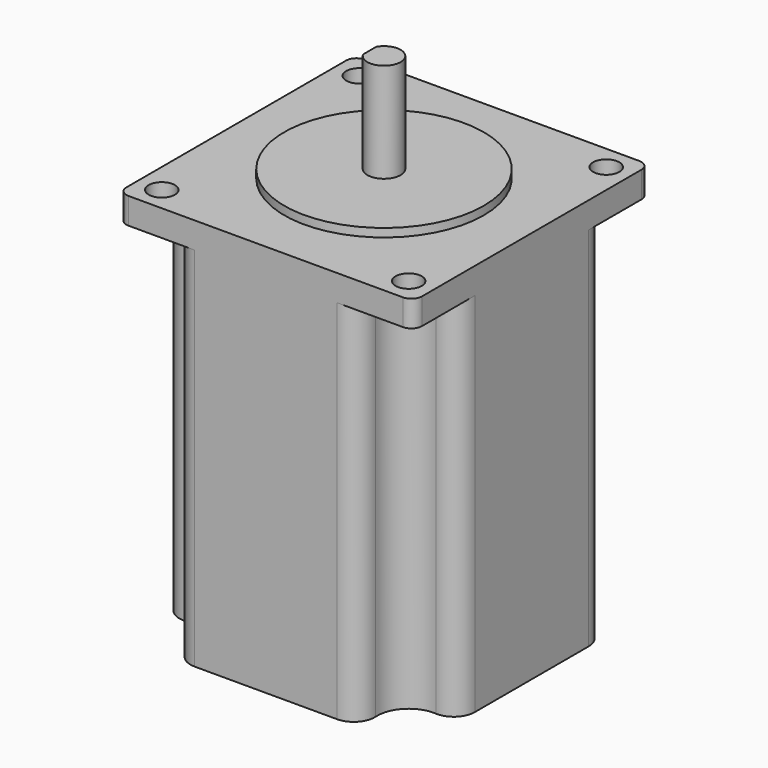
from build123d import *

# Parameters (mm, degrees)
F0_W      = 56.4
F0_H      = 56.4
F0_R      = 2.5
F1_DEPTH  = 75
F2_R      = 19.05
F3_DEPTH  = 1.6
F4_R      = 3.175
F5_DEPTH  = 19
F6_R      = 2.5
F7_DEPTH  = 2
F8_R      = 2
F10_DEPTH = 15.15
F11_R     = 2.5
F12_DEPTH = 70
F13_R     = 4


with BuildPart() as f1:
    # F0 (on Top) → F1 (new body)
    with BuildSketch(Plane.XY):
        Rectangle(F0_W, F0_H)
        with Locations((-23.57, -23.57)):
            Circle(F0_R, mode=Mode.SUBTRACT)
        with Locations((23.57, -23.57)):
            Circle(F0_R, mode=Mode.SUBTRACT)
        with Locations((-23.57, 23.57)):
            Circle(F0_R, mode=Mode.SUBTRACT)
        with Locations((23.57, 23.57)):
            Circle(F0_R, mode=Mode.SUBTRACT)
    extrude(amount=F1_DEPTH)

    # F2 (on face) → F3 (join)
    with BuildSketch(Plane.XY.offset(75)):
        Circle(F2_R)
    extrude(amount=F3_DEPTH)

    # F6 (on face) → F7 (join)
    with BuildSketch(Plane(origin=(-28.2, 0, 0), x_dir=(0, -1, 0), z_dir=(-1, 0, 0))):
        with Locations((0, 3.7299594842)):
            Circle(F6_R)
    extrude(amount=F7_DEPTH)

    # F8
    f8_edges = [f1.edges().sort_by_distance(p)[0] for p in [
        (-28.2, 28.2, 37.5),
        (28.2, 28.2, 37.5),
        (28.2, -28.2, 37.5),
        (-28.2, -28.2, 37.5),
    ]]
    fillet(f8_edges, radius=F8_R)

    # F11 (on face) → F12 (cut)
    with BuildSketch(Plane(origin=(0, 0, 0), x_dir=(1, 0, 0), z_dir=(0, 0, -1))):
        with BuildLine():
            ThreePointArc((-28.2, 19.7538370056), (-21.5426865067, 17.9228768386), (-17.57, 23.57))
            ThreePointArc((-17.57, 23.57), (-18.1433537997, 26.1295919629), (-19.7538370056, 28.2))
            Line((-19.7538370056, 28.2), (-26.2, 28.2))
            ThreePointArc((-26.2, 28.2), (-27.6142135624, 27.6142135624), (-28.2, 26.2))
            Line((-28.2, 26.2), (-28.2, 19.7538370056))
        make_face()
        with Locations((-23.57, 23.57)):
            Circle(F11_R, mode=Mode.SUBTRACT)
        with BuildLine():
            Line((26.2, 28.2), (19.7538370056, 28.2))
            ThreePointArc((19.7538370056, 28.2), (19.3273593129, 19.3273593129), (28.2, 19.7538370056))
            Line((28.2, 19.7538370056), (28.2, 26.2))
            ThreePointArc((28.2, 26.2), (27.6142135624, 27.6142135624), (26.2, 28.2))
        make_face()
        with Locations((23.57, 23.57)):
            Circle(F11_R, mode=Mode.SUBTRACT)
        with BuildLine():
            ThreePointArc((29.57, 23.57), (26.1295919629, 28.9966462003), (19.7538370056, 28.2))
            Line((19.7538370056, 28.2), (26.2, 28.2))
            ThreePointArc((26.2, 28.2), (27.6142135624, 27.6142135624), (28.2, 26.2))
            Line((28.2, 26.2), (28.2, 19.7538370056))
            ThreePointArc((28.2, 19.7538370056), (29.2171231614, 21.5426865067), (29.57, 23.57))
        make_face()
        with BuildLine():
            ThreePointArc((-17.57, -23.57), (-21.5426865067, -17.9228768386), (-28.2, -19.7538370056))
            Line((-28.2, -19.7538370056), (-28.2, -26.2))
            ThreePointArc((-28.2, -26.2), (-27.6142135624, -27.6142135624), (-26.2, -28.2))
            Line((-26.2, -28.2), (-19.7538370056, -28.2))
            ThreePointArc((-19.7538370056, -28.2), (-18.1433537997, -26.1295919629), (-17.57, -23.57))
        make_face()
        with Locations((-23.57, -23.57)):
            Circle(F11_R, mode=Mode.SUBTRACT)
        with BuildLine():
            Line((28.2, -26.2), (28.2, -19.7538370056))
            ThreePointArc((28.2, -19.7538370056), (19.3273593129, -19.3273593129), (19.7538370056, -28.2))
            Line((19.7538370056, -28.2), (26.2, -28.2))
            ThreePointArc((26.2, -28.2), (27.6142135624, -27.6142135624), (28.2, -26.2))
        make_face()
        with Locations((23.57, -23.57)):
            Circle(F11_R, mode=Mode.SUBTRACT)
        with Locations((-23.57, 23.57)):
            Circle(F11_R)
        with Locations((23.57, 23.57)):
            Circle(F11_R)
        with Locations((-23.57, -23.57)):
            Circle(F11_R)
        with Locations((23.57, -23.57)):
            Circle(F11_R)
    extrude(amount=-F12_DEPTH, mode=Mode.SUBTRACT)

    # F13
    f13_edges = [f1.edges().sort_by_distance(p)[0] for p in [
        (-28.2, 19.753837, 35),
        (-19.753837, 28.2, 35),
        (-28.2, -19.753837, 35),
        (-19.753837, -28.2, 35),
        (19.753837, -28.2, 35),
        (28.2, -19.753837, 35),
        (28.2, 19.753837, 35),
        (19.753837, 28.2, 35),
    ]]
    fillet(f13_edges, radius=F13_R)


with BuildPart() as f5:
    # F4 (on face) → F5 (new body)
    with BuildSketch(Plane.XY.offset(76.6)):
        Circle(F4_R)
    extrude(amount=F5_DEPTH)

    # F9 (on face) → F10 (cut)
    with BuildSketch(Plane.XY.offset(95.6)):
        with BuildLine():
            ThreePointArc((-2.745, 1.595493654), (-3.175, 0), (-2.745, -1.595493654))
            Line((-2.745, -1.595493654), (-2.745, 1.595493654))
        make_face()
    extrude(amount=-F10_DEPTH, mode=Mode.SUBTRACT)


solid = Compound([f1.part, f5.part])
